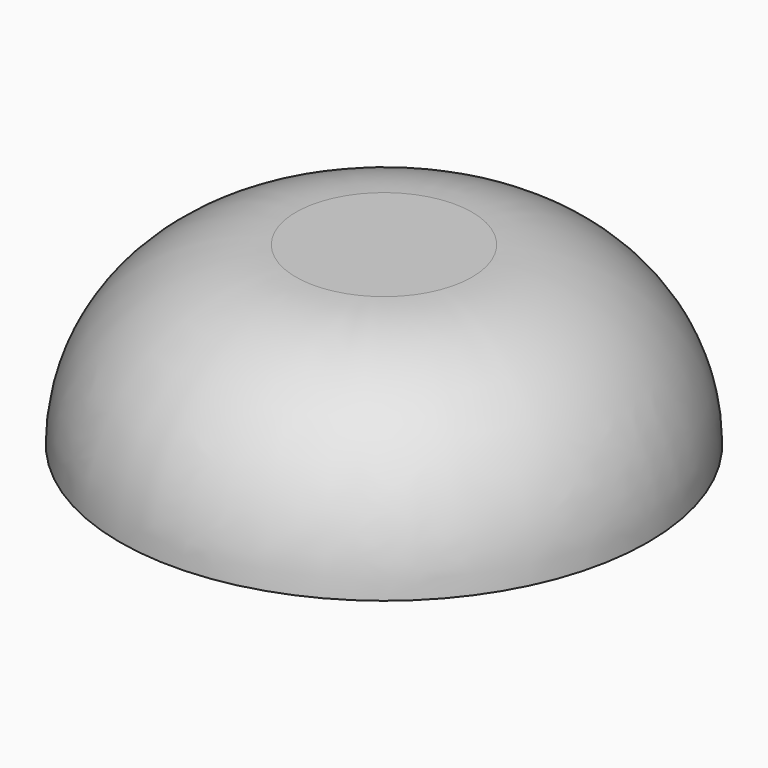
from build123d import *

# Parameters (mm, degrees)
F0_R     = 6.25
F0_R_2   = 3
F1_DEPTH = 3
F4_R     = 1
F5_DEPTH = 2


# Not quite as in the source:
# - a feature names something its author has since deleted; it is built from what else it names


with BuildPart() as f1:
    # F0 (on Top) → F1 (new body)
    with BuildSketch(Plane.XY):
        Circle(F0_R)
        Circle(F0_R_2, mode=Mode.SUBTRACT)
    extrude(amount=F1_DEPTH)

    # F2 (on Front) → F3 (revolve)
    with BuildSketch(Plane.XZ):
        with BuildLine():
            Line((5, 13), (0, 13))
            Line((0, 13), (0, 3))
            Line((0, 3), (15, 3))
            ThreePointArc((15, 3), (12.0710678119, 10.0710678119), (5, 13))
        make_face()
    revolve(axis=Axis((0, 0, 6.5), (0, 0, 1)))

    # F4
    f4_edges = [f1.edges().sort_by_distance(p)[0] for p in [
        (-6.25, 0, 0),
        (-6.25, 0, 3),
    ]]
    fillet(f4_edges, radius=F4_R)

    # F5 (cut): a face of the model
    f5_faces = [f1.faces().sort_by_distance(p)[0] for p in [
        (0, 0, 3),
    ]]
    extrude(f5_faces, amount=-F5_DEPTH, mode=Mode.SUBTRACT)


solid = f1.part
